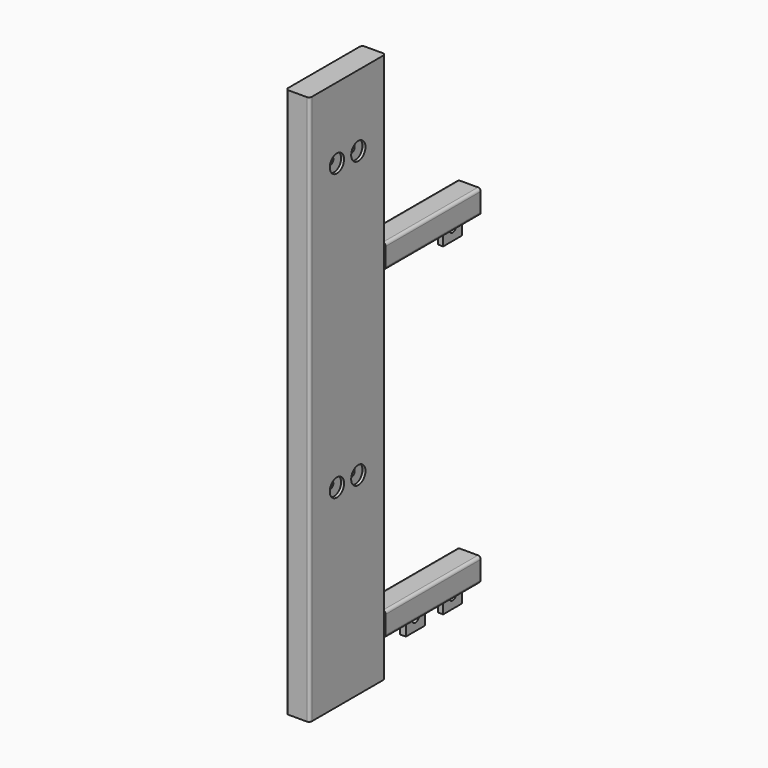
from build123d import *

# Parameters (mm, degrees)
F1_DEPTH  = 1168.4
F3_DEPTH  = 6.35
F5_START  = 1.27
F4_R      = 19.05
F5_DEPTH  = 22.225
F6_R      = 7.9375
F7_DEPTH  = 38.1
F8_R      = 7.9375
F9_DEPTH  = 38.1
F10_R     = 19.05
F11_DEPTH = 13.97
F12_W     = 12.7
F12_H     = 25.4
F13_DEPTH = 12.7
F14_R     = 8.6995
F15_DEPTH = 74.296
F17_DEPTH = 247.65
F19_DEPTH = 6.35
F21_DEPTH = 6.35
F22_W     = 50.8
F22_H     = 50.8
F22_R     = 9.652
F23_DEPTH = 11.1125
F24_R     = 8.5725
F25_DEPTH = 25.4
F26_W     = 50.8
F26_H     = 50.8
F26_R     = 9.652
F27_DEPTH = 12.7


with BuildPart() as f1:
    # F0 (on Top) → F1 (new body)
    with BuildSketch(Plane.XY):
        with BuildLine():
            Line((-19.431, -101.6), (19.431, -101.6))
            ThreePointArc((19.431, -101.6), (23.6517203769, -99.8517203769), (25.4, -95.631))
            Line((25.4, -95.631), (25.4, 95.631))
            ThreePointArc((25.4, 95.631), (23.6517203769, 99.8517203769), (19.431, 101.6))
            Line((19.431, 101.6), (-19.431, 101.6))
            ThreePointArc((-19.431, 101.6), (-23.6517203769, 99.8517203769), (-25.4, 95.631))
            Line((-25.4, 95.631), (-25.4, -95.631))
            ThreePointArc((-25.4, -95.631), (-23.6517203769, -99.8517203769), (-19.431, -101.6))
        make_face()
        with BuildLine():
            ThreePointArc((-15.875, -95.25), (-18.1200640303, -94.3200640303), (-19.05, -92.075))
            Line((-19.05, -92.075), (-19.05, 92.075))
            ThreePointArc((-19.05, 92.075), (-18.1200640303, 94.3200640303), (-15.875, 95.25))
            Line((-15.875, 95.25), (15.875, 95.25))
            ThreePointArc((15.875, 95.25), (18.1200640303, 94.3200640303), (19.05, 92.075))
            Line((19.05, 92.075), (19.05, -92.075))
            ThreePointArc((19.05, -92.075), (18.1200640303, -94.3200640303), (15.875, -95.25))
            Line((15.875, -95.25), (-15.875, -95.25))
        make_face(mode=Mode.SUBTRACT)
    extrude(amount=F1_DEPTH)

    # F2 (on face) → F3 (join)
    with BuildSketch(Plane.XY.offset(1168.4)):
        with BuildLine():
            Line((19.431, 101.6), (-19.431, 101.6))
            ThreePointArc((-19.431, 101.6), (-23.6517203769, 99.8517203769), (-25.4, 95.631))
            Line((-25.4, 95.631), (-25.4, -95.631))
            ThreePointArc((-25.4, -95.631), (-23.6517203769, -99.8517203769), (-19.431, -101.6))
            Line((-19.431, -101.6), (19.431, -101.6))
            ThreePointArc((19.431, -101.6), (23.6517203769, -99.8517203769), (25.4, -95.631))
            Line((25.4, -95.631), (25.4, 95.631))
            ThreePointArc((25.4, 95.631), (23.6517203769, 99.8517203769), (19.431, 101.6))
        make_face()
    extrude(amount=F3_DEPTH)

    # F10 (on face) → F11 (cut, through all)
    with BuildSketch(Plane.YZ.offset(11.43)):
        with Locations((-28.575, 1022.35)):
            Circle(F10_R)
        with Locations((28.575, 1022.35)):
            Circle(F10_R)
        with Locations((-28.575, 412.75)):
            Circle(F10_R)
        with Locations((28.575, 412.75)):
            Circle(F10_R)
    extrude(amount=F11_DEPTH, mode=Mode.SUBTRACT)

    # F12 (on face) → F13 (join)
    with BuildSketch(Plane(origin=(-25.4, 0, 0), x_dir=(0, -1, 0), z_dir=(-1, 0, 0))):
        with Locations((-34.925, 1060.45)):
            Rectangle(F12_W, F12_H)
        with Locations((-34.925, 450.85)):
            Rectangle(F12_W, F12_H)
    extrude(amount=F13_DEPTH)

    # F14 (on face) → F15 (cut, through all)
    with BuildSketch(Plane.YZ.offset(25.4)):
        with Locations((-28.575, 1022.35)):
            Circle(F14_R)
        with Locations((28.575, 1022.35)):
            Circle(F14_R)
        with Locations((28.575, 412.75)):
            Circle(F14_R)
        with Locations((-28.575, 412.75)):
            Circle(F14_R)
    extrude(amount=-F15_DEPTH, mode=Mode.SUBTRACT)

    # F16 (on face) → F17 (join)
    with BuildSketch(Plane(origin=(0, 101.6, 0), x_dir=(-1, 0, 0), z_dir=(0, 1, 0))):
        with BuildLine():
            Line((19.431, 819.15), (-19.431, 819.15))
            ThreePointArc((-19.431, 819.15), (-23.6517203769, 817.4017203769), (-25.4, 813.181))
            Line((-25.4, 813.181), (-25.4, 774.319))
            ThreePointArc((-25.4, 774.319), (-23.6517203769, 770.0982796231), (-19.431, 768.35))
            Line((-19.431, 768.35), (19.431, 768.35))
            ThreePointArc((19.431, 768.35), (23.6517203769, 770.0982796231), (25.4, 774.319))
            Line((25.4, 774.319), (25.4, 813.181))
            ThreePointArc((25.4, 813.181), (23.6517203769, 817.4017203769), (19.431, 819.15))
        make_face()
        with BuildLine():
            ThreePointArc((-19.05, 809.625), (-18.1200640303, 811.8700640303), (-15.875, 812.8))
            Line((-15.875, 812.8), (15.875, 812.8))
            ThreePointArc((15.875, 812.8), (18.1200640303, 811.8700640303), (19.05, 809.625))
            Line((19.05, 809.625), (19.05, 777.875))
            ThreePointArc((19.05, 777.875), (18.1200640303, 775.6299359697), (15.875, 774.7))
            Line((15.875, 774.7), (-15.875, 774.7))
            ThreePointArc((-15.875, 774.7), (-18.1200640303, 775.6299359697), (-19.05, 777.875))
            Line((-19.05, 777.875), (-19.05, 809.625))
        make_face(mode=Mode.SUBTRACT)
        with BuildLine():
            ThreePointArc((-19.431, 127), (-23.6517203769, 125.2517203769), (-25.4, 121.031))
            Line((-25.4, 121.031), (-25.4, 82.169))
            ThreePointArc((-25.4, 82.169), (-23.6517203769, 77.9482796231), (-19.431, 76.2))
            Line((-19.431, 76.2), (19.431, 76.2))
            ThreePointArc((19.431, 76.2), (23.6517203769, 77.9482796231), (25.4, 82.169))
            Line((25.4, 82.169), (25.4, 121.031))
            ThreePointArc((25.4, 121.031), (23.6517203769, 125.2517203769), (19.431, 127))
            Line((19.431, 127), (-19.431, 127))
        make_face()
        with BuildLine():
            Line((-19.05, 85.725), (-19.05, 117.475))
            ThreePointArc((-19.05, 117.475), (-18.1200640303, 119.7200640303), (-15.875, 120.65))
            Line((-15.875, 120.65), (15.875, 120.65))
            ThreePointArc((15.875, 120.65), (18.1200640303, 119.7200640303), (19.05, 117.475))
            Line((19.05, 117.475), (19.05, 85.725))
            ThreePointArc((19.05, 85.725), (18.1200640303, 83.4799359697), (15.875, 82.55))
            Line((15.875, 82.55), (-15.875, 82.55))
            ThreePointArc((-15.875, 82.55), (-18.1200640303, 83.4799359697), (-19.05, 85.725))
        make_face(mode=Mode.SUBTRACT)
    extrude(amount=F17_DEPTH)

    # F18 (on face) → F19 (join)
    with BuildSketch(Plane(origin=(0, 349.25, 0), x_dir=(-1, 0, 0), z_dir=(0, 1, 0))):
        with BuildLine():
            Line((19.431, 819.15), (-19.431, 819.15))
            ThreePointArc((-19.431, 819.15), (-23.6517203769, 817.4017203769), (-25.4, 813.181))
            Line((-25.4, 813.181), (-25.4, 774.319))
            ThreePointArc((-25.4, 774.319), (-23.6517203769, 770.0982796231), (-19.431, 768.35))
            Line((-19.431, 768.35), (19.431, 768.35))
            ThreePointArc((19.431, 768.35), (23.6517203769, 770.0982796231), (25.4, 774.319))
            Line((25.4, 774.319), (25.4, 813.181))
            ThreePointArc((25.4, 813.181), (23.6517203769, 817.4017203769), (19.431, 819.15))
        make_face()
    extrude(amount=F19_DEPTH)

    # F20 (on face) → F21 (join)
    with BuildSketch(Plane(origin=(0, 349.25, 0), x_dir=(-1, 0, 0), z_dir=(0, 1, 0))):
        with BuildLine():
            Line((19.431, 127), (-19.431, 127))
            ThreePointArc((-19.431, 127), (-23.6517203769, 125.2517203769), (-25.4, 121.031))
            Line((-25.4, 121.031), (-25.4, 82.169))
            ThreePointArc((-25.4, 82.169), (-23.6517203769, 77.9482796231), (-19.431, 76.2))
            Line((-19.431, 76.2), (19.431, 76.2))
            ThreePointArc((19.431, 76.2), (23.6517203769, 77.9482796231), (25.4, 82.169))
            Line((25.4, 82.169), (25.4, 121.031))
            ThreePointArc((25.4, 121.031), (23.6517203769, 125.2517203769), (19.431, 127))
        make_face()
    extrude(amount=F21_DEPTH)

    # F22 (on face) → F23 (join)
    with BuildSketch(Plane(origin=(-25.4, 0, 0), x_dir=(0, -1, 0), z_dir=(-1, 0, 0))):
        with Locations((-330.2, 742.95)):
            Rectangle(F22_W, F22_H)
        with Locations((-330.2, 742.95)):
            Circle(F22_R, mode=Mode.SUBTRACT)
        with Locations((-330.2, 50.8)):
            Rectangle(F22_W, F22_H)
        with Locations((-330.2, 50.8)):
            Circle(F22_R, mode=Mode.SUBTRACT)
    extrude(amount=-F23_DEPTH)

    # F24 (on face) → F25 (cut)
    with BuildSketch(Plane(origin=(-25.4, 0, 0), x_dir=(0, -1, 0), z_dir=(-1, 0, 0))):
        with Locations((-50.8, 1111.25)):
            Circle(F24_R)
        with Locations((-50.8, 501.65)):
            Circle(F24_R)
    extrude(amount=-F25_DEPTH, mode=Mode.SUBTRACT)

    # F26 (on face) → F27 (join)
    with BuildSketch(Plane(origin=(-25.4, 0, 0), x_dir=(0, -1, 0), z_dir=(-1, 0, 0))):
        with Locations((-228.6, 50.8)):
            Rectangle(F26_W, F26_H)
        with Locations((-228.6, 50.8)):
            Circle(F26_R, mode=Mode.SUBTRACT)
    extrude(amount=-F27_DEPTH)


with BuildPart() as f5:
    # F4 (on face) → F5 (new body)
    with BuildSketch(Plane(origin=(-25.4, 0, 0), x_dir=(0, -1, 0), z_dir=(-1, 0, 0)).offset(F5_START)):
        with Locations((28.575, 1022.35)):
            Circle(F4_R)
    extrude(amount=F5_DEPTH)

    # F6 (on face) → F7 (join)
    with BuildSketch(Plane.YZ.offset(-26.67)):
        with Locations((-28.575, 1022.35)):
            Circle(F6_R)
    extrude(amount=F7_DEPTH)


with BuildPart() as f5b:
    # F4 (on face) → F5, piece 2 (new body)
    with BuildSketch(Plane(origin=(-25.4, 0, 0), x_dir=(0, -1, 0), z_dir=(-1, 0, 0)).offset(F5_START)):
        with Locations((-28.575, 1022.35)):
            Circle(F4_R)
    extrude(amount=F5_DEPTH)

    # F8 (on face) → F9 (join)
    with BuildSketch(Plane.YZ.offset(-26.67)):
        with Locations((28.575, 1022.35)):
            Circle(F8_R)
    extrude(amount=F9_DEPTH)


with BuildPart() as f5c:
    # F4 (on face) → F5, piece 3 (new body)
    with BuildSketch(Plane(origin=(-25.4, 0, 0), x_dir=(0, -1, 0), z_dir=(-1, 0, 0)).offset(F5_START)):
        with Locations((-28.575, 412.75)):
            Circle(F4_R)
    extrude(amount=F5_DEPTH)


with BuildPart() as f5d:
    # F4 (on face) → F5, piece 4 (new body)
    with BuildSketch(Plane(origin=(-25.4, 0, 0), x_dir=(0, -1, 0), z_dir=(-1, 0, 0)).offset(F5_START)):
        with Locations((28.575, 412.75)):
            Circle(F4_R)
    extrude(amount=F5_DEPTH)


with BuildPart() as f7:
    # F6 (on face) → F7, piece 2 (new body)
    with BuildSketch(Plane.YZ.offset(-26.67)):
        with Locations((-28.575, 412.75)):
            Circle(F6_R)
    extrude(amount=F7_DEPTH)


with BuildPart() as f9:
    # F8 (on face) → F9, piece 2 (new body)
    with BuildSketch(Plane.YZ.offset(-26.67)):
        with Locations((28.575, 412.75)):
            Circle(F8_R)
    extrude(amount=F9_DEPTH)


solid = Compound([f1.part, f5.part, f5b.part, f5c.part, f5d.part, f7.part, f9.part])
